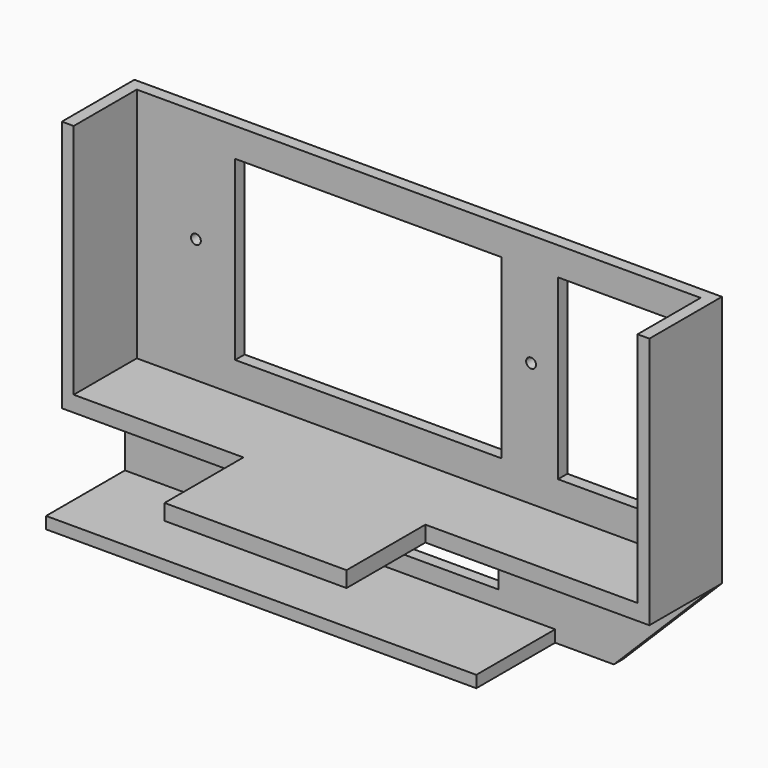
from build123d import *

# Parameters (mm, degrees)
F0_W         = 147
F0_H         = 60
F1_DEPTH     = 3
F2_W         = 3
F2_H         = 60
F3_DEPTH     = 20
F4_DEPTH     = 4
F5_W         = 141
F5_H         = 4
F6_DEPTH     = 20
F7_DEPTH     = 2
F8_DEPTH     = 2
F10_W        = 5
F10_H        = 11.305693537
F11_DEPTH    = 15
F9_R         = 1.25
F12_DEPTH    = 25
F13_T4_DEPTH = 82.150489639
F13_T9_DEPTH = 82.150489639
F14_W        = 14.2459415197
F14_H        = 3
F14_W_2      = 46.2986054569
F14_W_3      = 5
F14_W_4      = 78.4554530233
F15_DEPTH    = 25
F16_SIZE     = 25
F17_W        = 109.1084168532
F17_H        = 3
F18_DEPTH    = 25
F19_W        = 67.5222836435
F19_H        = 44.9108928442
F19_W_2      = 29.4727757573
F19_H_2      = 45.0668334961
F20_DEPTH    = 25
F21_W        = 65.4478734359
F21_H        = 13.5871618986
F22_DEPTH    = 25
F23_W        = 46.1584180593
F23_H        = 4
F24_DEPTH    = 25


# Not quite as in the source:
# - a fillet or chamfer that OpenCascade refuses, or shapes differently, is made with other operations: its cross-section is extruded or revolved along the edge and cut away or added


with BuildPart() as f1:
    # F0 (on Front) → F1 (new body)
    with BuildSketch(Plane.XZ):
        with Locations((39.3571183681, 3.4620302916)):
            Rectangle(F0_W, F0_H)
    extrude(amount=F1_DEPTH)

    # F2 (on face) → F3 (join)
    with BuildSketch(Plane.XZ.offset(3)):
        with Locations((-32.6428816319, 3.4620302916)):
            Rectangle(F2_W, F2_H)
        with Locations((111.3571183681, 3.4620302916)):
            Rectangle(F2_W, F2_H)
    extrude(amount=F3_DEPTH)

    # F4 (add): a face of the model
    f4_faces = [f1.faces().sort_by_distance(p)[0] for p in [
        (-32.6549972277, -11.5, -26.5379697084),
    ]]
    extrude(f4_faces, amount=F4_DEPTH)

    # F5 (on face) → F6 (join)
    with BuildSketch(Plane.XZ.offset(3)):
        with Locations((39.3571183681, -28.5379697084)):
            Rectangle(F5_W, F5_H)
    extrude(amount=F6_DEPTH)

    # F7 (add): a face of the model
    f7_faces = [f1.faces().sort_by_distance(p)[0] for p in [
        (112.8571183681, -11.5, 1.4620302916),
    ]]
    extrude(f7_faces, amount=F7_DEPTH)

    # F8 (cut): a face of the model
    f8_faces = [f1.faces().sort_by_distance(p)[0] for p in [
        (109.8571183681, -13, 3.4620302916),
    ]]
    extrude(f8_faces, amount=-F8_DEPTH, mode=Mode.SUBTRACT)

    # F10 (on face) → F11 (join)
    with BuildSketch(Plane(origin=(0, 0, -30.5379697084), x_dir=(1, 0, 0), z_dir=(0, 0, -1))):
        with Locations((-17.3969401121, 5.6528467685)):
            Rectangle(F10_W, F10_H)
        with Locations((66.0585129112, 5.6528467685)):
            Rectangle(F10_W, F10_H)
    extrude(amount=F11_DEPTH)

    # F9 (on face) → F12 (cut)
    with BuildSketch(Plane.XZ.offset(3)):
        with Locations((-16.1428816319, 4.912131466)):
            Circle(F9_R)
        with Locations((68.8571183681, 4.912131466)):
            Circle(F9_R)
    extrude(amount=-F12_DEPTH, mode=Mode.SUBTRACT)

    # F13: chamfer of 15 on 2 edges, made by hand


with BuildPart() as f13_tool2:
    # F13_s3 → F13_t4 (new body)
    with BuildSketch(Plane.YZ.offset(23.6783047074)):
        Polygon((3.694306463, -45.5379697084), (-11.305693537, -30.5379697084), (-11.305693537, -45.5379697084), align=None)
    extrude(amount=-F13_T4_DEPTH)

    split(bisect_by=Plane.XY.offset(-30.5379697084), keep=Keep.BOTTOM)


with BuildPart() as f1_1:
    add(f1.part)

    # F13_t1: cut F13_tool2
    add(f13_tool2.part, mode=Mode.SUBTRACT)


with BuildPart() as f13_tool7:
    # F13_s8 → F13_t9 (new body)
    with BuildSketch(Plane.YZ.offset(107.1337577307)):
        Polygon((3.694306463, -45.5379697084), (-11.305693537, -30.5379697084), (-11.305693537, -45.5379697084), align=None)
    extrude(amount=-F13_T9_DEPTH)

    split(bisect_by=Plane.XY.offset(-30.5379697084), keep=Keep.BOTTOM)


with BuildPart() as f1_2:
    add(f1_1.part)

    # F13_t6: cut F13_tool7
    add(f13_tool7.part, mode=Mode.SUBTRACT)

    # F14 (on face) → F15 (join)
    with BuildSketch(Plane(origin=(0, 0, -30.5379697084), x_dir=(1, 0, 0), z_dir=(0, 0, -1))):
        with Locations((-27.019910872, 1.5)):
            Rectangle(F14_W, F14_H)
        with Locations((91.7078156397, 1.5)):
            Rectangle(F14_W_2, F14_H)
        with Locations((-17.3969401121, 1.5)):
            Rectangle(F14_W_3, F14_H)
        with Locations((66.0585129112, 1.5)):
            Rectangle(F14_W_3, F14_H)
        with Locations((24.3307863995, 1.5)):
            Rectangle(F14_W_4, F14_H)
    extrude(amount=F15_DEPTH)

    # F16
    f16_edges = [f1_2.edges().sort_by_distance(p)[0] for p in [
        (114.857118, -1.5, -55.53797),
    ]]
    chamfer(f16_edges, length=F16_SIZE)

    # F17 (on face) → F18 (join)
    with BuildSketch(Plane.XZ.offset(3)):
        with Locations((20.4113267948, -54.0379697084)):
            Rectangle(F17_W, F17_H)
    extrude(amount=F18_DEPTH)

    # F19 (on face) → F20 (cut)
    with BuildSketch(Plane.XZ.offset(3)):
        with Locations((27.5696460158, 3.6646034569)):
            Rectangle(F19_W, F19_H)
        with Locations((90.4137082398, 3.7425737828)):
            Rectangle(F19_W_2, F19_H_2)
    extrude(amount=-F20_DEPTH, mode=Mode.SUBTRACT)

    # F21 (on face) → F22 (cut)
    with BuildSketch(Plane.XZ.offset(3)):
        with Locations((27.9176128097, -41.5276624262)):
            Rectangle(F21_W, F21_H)
    extrude(amount=-F22_DEPTH, mode=Mode.SUBTRACT)

    # F23 (on face) → F24 (join)
    with BuildSketch(Plane.XZ.offset(23)):
        with Locations((34.9768251181, -28.5379697084)):
            Rectangle(F23_W, F23_H)
    extrude(amount=F24_DEPTH)


solid = f1_2.part
